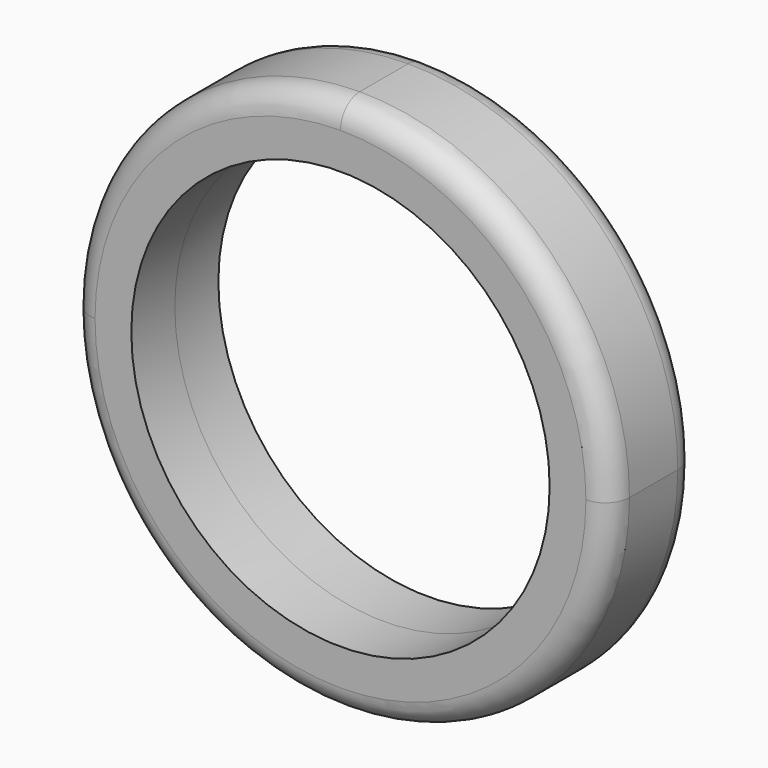
from build123d import *

# Parameters (mm, degrees)
F0_R          = 8.65
F1_DEPTH      = 2.25
F1_DEPTH_BACK = 2.25
F2_R          = 1


with BuildPart() as f1:
    # F0 (on Front) → F1 (new body, two sides)
    with BuildSketch(Plane.XZ) as f1_sk:
        with BuildLine():
            ThreePointArc((-11.15, 0), (0, -11.15), (11.15, 0))
            ThreePointArc((11.15, 0), (7.884241, 7.884241), (0, 11.15))
            ThreePointArc((0, 11.15), (-7.884241, 7.884241), (-11.15, 0))
        make_face()
        Circle(F0_R, mode=Mode.SUBTRACT)
    extrude(amount=F1_DEPTH)
    extrude(f1_sk.sketch, amount=-F1_DEPTH_BACK)

    # F2
    f2_edges = [f1.edges().sort_by_distance(p)[0] for p in [
        (-11.15, -2.25, 0),
        (-11.15, 2.25, 0),
    ]]
    fillet(f2_edges, radius=F2_R)


solid = f1.part
